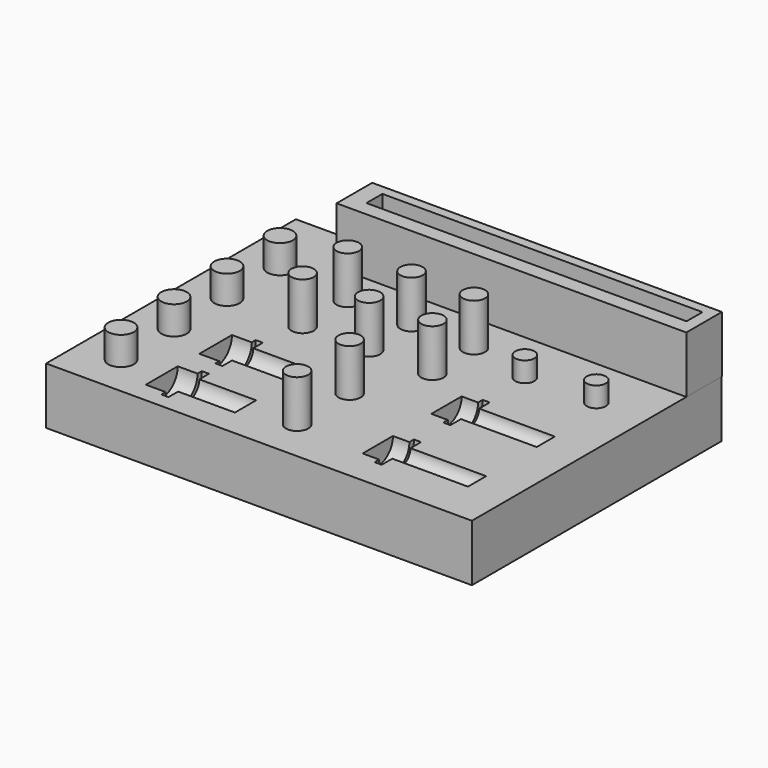
from build123d import *

# Parameters (mm, degrees)
F0_W      = 225
F0_H      = 165
F1_DEPTH  = 30
F2_R      = 6.75
F3_DEPTH  = 15
F5_W      = 0.0118811131
F5_H      = 10.5422940105
F5_W_2    = 10.4881188869
F5_W_3    = 30
F5_H_2    = 7
F10_R     = 5.9
F11_DEPTH = 12.85
F12_DEPTH = 25
F15_W     = 8.7
F15_H     = 10
F15_W_2   = 40
F15_H_2   = 6
F17_R     = 5.05
F18_DEPTH = 10.6
F19_W     = 184.7800500691
F19_H     = 23.5
F20_DEPTH = 30
F21_W     = 169.1280193627
F21_H     = 10.5079561472
F22_DEPTH = 50


# Not quite as in the source:
# - a feature names something its author has since deleted; it is built from what else it names


with BuildPart() as f1:
    # F0 (on Top) → F1 (new body)
    with BuildSketch(Plane.XY):
        with Locations((112.5, 82.5)):
            Rectangle(F0_W, F0_H)
    extrude(amount=F1_DEPTH)

    # F2 (on face) → F3 (join)
    with BuildSketch(Plane.XY.offset(30)):
        with Locations((22, 127)):
            Circle(F2_R)
        with Locations((22, 92)):
            Circle(F2_R)
        with Locations((22, 57)):
            Circle(F2_R)
        with Locations((22, 22)):
            Circle(F2_R)
    extrude(amount=F3_DEPTH)

    # F5 (on face) → F6 (revolve, cut)
    with BuildSketch(Plane.XY.offset(30)):
        with Locations((43.9940594435, 16.1421531811)):
            Rectangle(F5_W, F5_H)
        with Locations((49.2440594435, 16.1421531811)):
            Rectangle(F5_W_2, F5_H)
        Polygon((58.2381188869, 21.4133001864), (54.4881188869, 21.4133001864), (54.4881188869, 10.8710061759), (54.4881188869, 8.0633001864), (58.2381188869, 8.0633001864), (58.2381188869, 14.4133001864), align=None)
        with Locations((73.2381188869, 17.9133001864)):
            Rectangle(F5_W_3, F5_H_2)
    revolve(axis=Axis((49.2381188869, 21.4133001864, 30), (1, 0, 0)), mode=Mode.SUBTRACT)

    # F7 (on face) → F8 (revolve, cut)
    with BuildSketch(Plane.XY.offset(30)):
        Polygon((44, 57), (44, 46.25), (54.5, 46.25), (54.5, 43.65), (58.25, 43.65), (58.25, 50), (88.25, 50), (88.25, 57), (58.25, 57), (54.5, 57), align=None)
    revolve(axis=Axis((49.25, 57, 30), (1, 0, 0)), mode=Mode.SUBTRACT)

    # F10 (on face) → F11 (join)
    with BuildSketch(Plane.XY.offset(30)):
        with Locations((62.1212087572, 121.5757578611)):
            Circle(F10_R)
        with Locations((62.1212087572, 91.7575731874)):
            Circle(F10_R)
    extrude(amount=F11_DEPTH)

    # F10 (on face) → F12 (join)
    with BuildSketch(Plane.XY.offset(30)):
        with Locations((62.1212087572, 121.5757578611)):
            Circle(F10_R)
        with Locations((62.1212087572, 91.7575731874)):
            Circle(F10_R)
        with Locations((96.6326966882, 92.5912261009)):
            Circle(F10_R)
        with Locations((96.1869060993, 121.1215853691)):
            Circle(F10_R)
        with Locations((114.9099543691, 22.1569109708)):
            Circle(F10_R)
        with Locations((129.1751265526, 121.1215853691)):
            Circle(F10_R)
        with Locations((130.0667077303, 92.5912261009)):
            Circle(F10_R)
        with Locations((114.4641637802, 57.3740676045)):
            Circle(F10_R)
    extrude(amount=F12_DEPTH)

    # F13 (on face) → F14 (revolve, cut)
    with BuildSketch(Plane.XY.offset(30)):
        Polygon((160.9424221039, 28.7878794968), (152.2424221039, 28.7878794968), (152.2424221039, 18.7878794968), (160.9424221039, 18.7878794968), (160.9424221039, 15.7878794968), (164.6924221039, 15.7878794968), (164.6924221039, 22.7878794968), (204.6924221039, 22.7878794968), (204.6924221039, 28.7878794968), (164.6924221039, 28.7878794968), align=None)
    revolve(axis=Axis((184.6924221039, 28.7878794968, 30), (1, 0, 0)), mode=Mode.SUBTRACT)

    # F15 (on face) → F16 (revolve, cut)
    with BuildSketch(Plane.XY.offset(30)):
        with Locations((156.6197043896, 69.1212128103)):
            Rectangle(F15_W, F15_H)
        Polygon((164.7197043896, 74.1212128103), (160.9697043896, 74.1212128103), (160.9697043896, 64.1212128103), (160.9697043896, 61.1212128103), (164.7197043896, 61.1212128103), (164.7197043896, 68.1212128103), align=None)
        with Locations((184.7197043896, 71.1212128103)):
            Rectangle(F15_W_2, F15_H_2)
    revolve(axis=Axis((184.7197043896, 74.1212128103, 30), (1, 0, 0)), mode=Mode.SUBTRACT)

    # F17 (on face) → F18 (join)
    with BuildSketch(Plane.XY.offset(30)):
        with Locations((162.1633470058, 113.5432049632)):
            Circle(F17_R)
        with Locations((199.1636604071, 114.4347786903)):
            Circle(F17_R)
    extrude(amount=F18_DEPTH)

    # F19 (on face) → F20 (join)
    with BuildSketch(Plane.XY.offset(30)):
        with Locations((132.609969005, 153.3750020266)):
            Rectangle(F19_W, F19_H)
    extrude(amount=F20_DEPTH)

    # F21 (on face) → F22 (cut)
    with BuildSketch(Plane.XY.offset(60)):
        with Locations((134.2664714903, 154.7421440482)):
            Rectangle(F21_W, F21_H)
    extrude(amount=-F22_DEPTH, mode=Mode.SUBTRACT)


solid = f1.part
